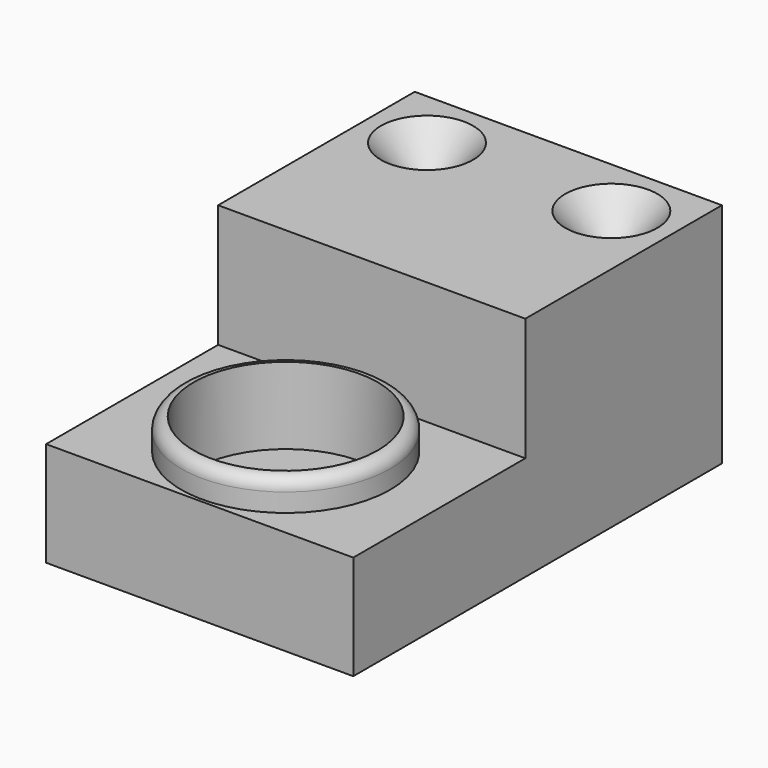
from build123d import *

# Parameters (mm, degrees)
F1_DEPTH       = 63.5
F2_R           = 19.05
F3_DEPTH       = 9.525
F4_R           = 21.59
F4_R_2         = 19.05
F5_DEPTH       = 6.35
F6_R           = 2.53999
F8_D           = 6.35
F8_CSINK_D     = 19.05
F8_CSINK_ANGLE = 82


# Not quite as in the source:
# - a fillet or chamfer is up to 0.001 mm smaller than in the source, because OpenCascade refuses the exact size


with BuildPart() as f1:
    # F0 (on Right) → F1 (new body)
    with BuildSketch(Plane.YZ):
        Polygon((0, 21.59), (0, 0), (95.25, 0), (95.25, 46.99), (44.45, 46.99), (44.45, 21.59), align=None)
    extrude(amount=-F1_DEPTH)

    # F2 (on face) → F3 (cut)
    with BuildSketch(Plane.XY.offset(21.59)):
        with Locations((-31.75, 22.225)):
            Circle(F2_R)
    extrude(amount=-F3_DEPTH, mode=Mode.SUBTRACT)

    # F4 (on face) → F5 (join)
    with BuildSketch(Plane.XY.offset(21.59)):
        with Locations((-31.75, 22.225)):
            Circle(F4_R)
        with Locations((-31.75, 22.225)):
            Circle(F4_R_2, mode=Mode.SUBTRACT)
    extrude(amount=F5_DEPTH)

    # F6 (radius 2.54 in the source; OpenCascade refuses exactly that, so slightly less here)
    f6_edges = [f1.edges().sort_by_distance(p)[0] for p in [
        (-53.34, 22.225, 27.94),
    ]]
    fillet(f6_edges, radius=F6_R)

    # F8 (through all)
    with Locations(Plane.XY.offset(46.99)):
        with Locations((-50.8, 82.55), (-12.7, 82.55)):
            CounterSinkHole(F8_D / 2, F8_CSINK_D / 2, counter_sink_angle=F8_CSINK_ANGLE)


solid = f1.part
